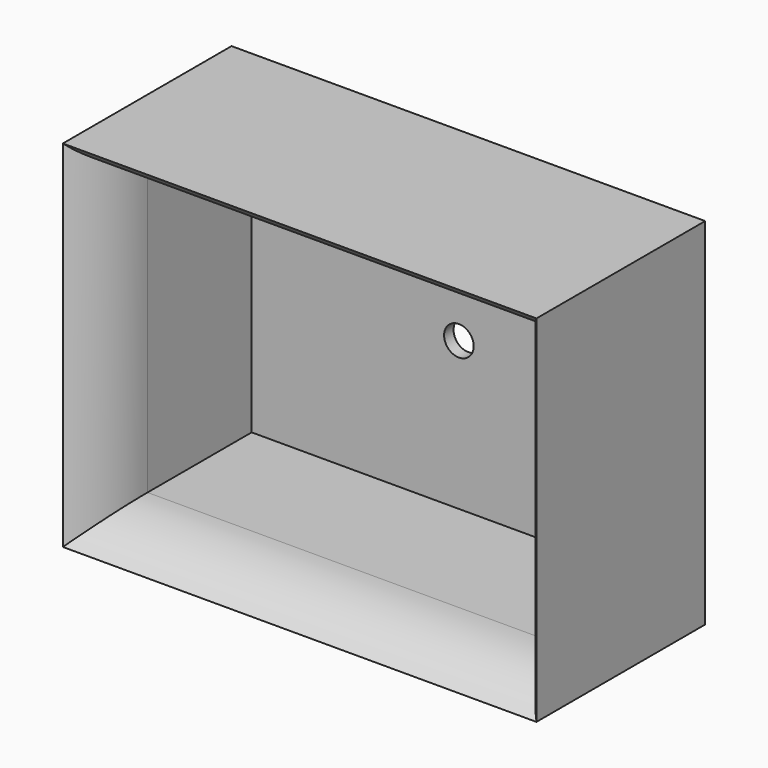
from build123d import *

# Parameters (mm, degrees)
F0_W         = 101.6
F0_H         = 76.2
F0_W_2       = 88.9
F0_H_2       = 63.5
F1_DEPTH     = 50.8
F2_DEPTH     = 2.54
F3_T1_DEPTH  = 63.5
F3_T3_DEPTH  = 88.9
F3_T9_DEPTH  = 139.7
F3_T15_DEPTH = 114.3
F3_T24_DEPTH = 139.7
F3_T30_DEPTH = 114.3
F3_T39_DEPTH = 139.7
F3_T45_DEPTH = 114.3
F3_T54_DEPTH = 114.3
F3_T60_DEPTH = 139.7
F4_R         = 3.175
F5_DEPTH     = 2.541


# Not quite as in the source:
# - a fillet or chamfer that OpenCascade refuses, or shapes differently, is made with other operations: its cross-section is extruded or revolved along the edge and cut away or added


with BuildPart() as f1:
    # F0 (on Front) → F1 (new body)
    with BuildSketch(Plane.XZ):
        Rectangle(F0_W, F0_H)
        Rectangle(F0_W_2, F0_H_2, mode=Mode.SUBTRACT)
    extrude(amount=F1_DEPTH)

    # F3: fillet of radius 20.32 on 4 edges, made by hand

    # F3_s2 → F3_t1 (cut)
    with BuildSketch(Plane.XY.offset(-31.75)):
        with BuildLine():
            ThreePointArc((-44.45, -30.48), (-50.4015902063, -44.8484097937), (-64.77, -50.8))
            Line((-64.77, -50.8), (-44.45, -50.8))
            Line((-44.45, -50.8), (-44.45, -30.48))
        make_face()
        with BuildLine():
            ThreePointArc((44.45, -30.48), (50.4015902063, -44.8484097937), (64.77, -50.8))
            Line((64.77, -50.8), (44.45, -50.8))
            Line((44.45, -50.8), (44.45, -30.48))
        make_face()
    extrude(amount=F3_T1_DEPTH, mode=Mode.SUBTRACT)

    # F3_s4 → F3_t3 (cut)
    with BuildSketch(Plane.YZ.offset(-44.45)):
        with BuildLine():
            ThreePointArc((-30.48, 31.75), (-44.8484097937, 37.7015902063), (-50.8, 52.07))
            Line((-50.8, 52.07), (-50.8, 31.75))
            Line((-50.8, 31.75), (-30.48, 31.75))
        make_face()
        with BuildLine():
            ThreePointArc((-30.48, -31.75), (-44.8484097937, -37.7015902063), (-50.8, -52.07))
            Line((-50.8, -52.07), (-50.8, -31.75))
            Line((-50.8, -31.75), (-30.48, -31.75))
        make_face()
    extrude(amount=F3_T3_DEPTH, mode=Mode.SUBTRACT)


with BuildPart() as f2:
    # F0 (on Front) → F2 (new body)
    with BuildSketch(Plane.XZ):
        Rectangle(F0_W_2, F0_H_2)
    extrude(amount=F2_DEPTH)

    # F4 (on face) → F5 (cut, through all)
    with BuildSketch(Plane.XZ.offset(2.54)):
        Circle(F4_R)
    extrude(amount=-F5_DEPTH, mode=Mode.SUBTRACT)


with BuildPart() as f3_tool7:
    # F3_s8 → F3_t9 (new body)
    with BuildSketch(Plane.YZ.offset(44.45)):
        with BuildLine():
            ThreePointArc((-30.48, -31.75), (-44.8484097937, -37.7015902063), (-50.8, -52.07))
            Line((-50.8, -52.07), (-50.8, -31.75))
            Line((-50.8, -31.75), (-30.48, -31.75))
        make_face()
    extrude(amount=-F3_T9_DEPTH)

    split(bisect_by=Plane.YZ.offset(-50.8), keep=Keep.TOP)

    split(bisect_by=Plane.XY.offset(-38.1), keep=Keep.TOP)

    split(bisect_by=Plane.YZ.offset(-44.45), keep=Keep.BOTTOM)


with BuildPart() as f3_tool13:
    # F3_s14 → F3_t15 (new body)
    with BuildSketch(Plane.XY.offset(-82.55)):
        with BuildLine():
            ThreePointArc((-44.45, -30.48), (-50.4015902063, -44.8484097937), (-64.77, -50.8))
            Line((-64.77, -50.8), (-44.45, -50.8))
            Line((-44.45, -50.8), (-44.45, -30.48))
        make_face()
    extrude(amount=F3_T15_DEPTH)

    split(bisect_by=Plane.YZ.offset(-50.8), keep=Keep.TOP)

    split(bisect_by=Plane.XY.offset(-38.1), keep=Keep.TOP)

    split(bisect_by=Plane.XY.offset(-31.75), keep=Keep.BOTTOM)


with BuildPart() as f3_tool7_1:
    add(f3_tool7.part)

    # F3_t19: intersect F3_tool13
    add(f3_tool13.part, mode=Mode.INTERSECT)


with BuildPart() as f1_1:
    add(f1.part)

    # F3_t5: cut F3_tool7
    add(f3_tool7_1.part, mode=Mode.SUBTRACT)


with BuildPart() as f3_tool22:
    # F3_s23 → F3_t24 (new body)
    with BuildSketch(Plane.YZ.offset(-95.25)):
        with BuildLine():
            ThreePointArc((-30.48, 31.75), (-44.8484097937, 37.7015902063), (-50.8, 52.07))
            Line((-50.8, 52.07), (-50.8, 31.75))
            Line((-50.8, 31.75), (-30.48, 31.75))
        make_face()
    extrude(amount=F3_T24_DEPTH)

    split(bisect_by=Plane.XY.offset(38.1), keep=Keep.BOTTOM)

    split(bisect_by=Plane.YZ.offset(-50.8), keep=Keep.TOP)

    split(bisect_by=Plane.YZ.offset(-44.45), keep=Keep.BOTTOM)


with BuildPart() as f3_tool28:
    # F3_s29 → F3_t30 (new body)
    with BuildSketch(Plane.XY.offset(-31.75)):
        with BuildLine():
            ThreePointArc((-44.45, -30.48), (-50.4015902063, -44.8484097937), (-64.77, -50.8))
            Line((-64.77, -50.8), (-44.45, -50.8))
            Line((-44.45, -50.8), (-44.45, -30.48))
        make_face()
    extrude(amount=F3_T30_DEPTH)

    split(bisect_by=Plane.XY.offset(38.1), keep=Keep.BOTTOM)

    split(bisect_by=Plane.YZ.offset(-50.8), keep=Keep.TOP)

    split(bisect_by=Plane.XY.offset(31.75), keep=Keep.TOP)


with BuildPart() as f3_tool22_1:
    add(f3_tool22.part)

    # F3_t34: intersect F3_tool28
    add(f3_tool28.part, mode=Mode.INTERSECT)


with BuildPart() as f1_2:
    add(f1_1.part)

    # F3_t20: cut F3_tool22
    add(f3_tool22_1.part, mode=Mode.SUBTRACT)


with BuildPart() as f3_tool37:
    # F3_s38 → F3_t39 (new body)
    with BuildSketch(Plane.YZ.offset(-44.45)):
        with BuildLine():
            ThreePointArc((-30.48, 31.75), (-44.8484097937, 37.7015902063), (-50.8, 52.07))
            Line((-50.8, 52.07), (-50.8, 31.75))
            Line((-50.8, 31.75), (-30.48, 31.75))
        make_face()
    extrude(amount=F3_T39_DEPTH)

    split(bisect_by=Plane.YZ.offset(50.8), keep=Keep.BOTTOM)

    split(bisect_by=Plane.XY.offset(38.1), keep=Keep.BOTTOM)

    split(bisect_by=Plane.YZ.offset(44.45), keep=Keep.TOP)


with BuildPart() as f3_tool43:
    # F3_s44 → F3_t45 (new body)
    with BuildSketch(Plane.XY.offset(82.55)):
        with BuildLine():
            ThreePointArc((44.45, -30.48), (50.4015902063, -44.8484097937), (64.77, -50.8))
            Line((64.77, -50.8), (44.45, -50.8))
            Line((44.45, -50.8), (44.45, -30.48))
        make_face()
    extrude(amount=-F3_T45_DEPTH)

    split(bisect_by=Plane.YZ.offset(50.8), keep=Keep.BOTTOM)

    split(bisect_by=Plane.XY.offset(38.1), keep=Keep.BOTTOM)

    split(bisect_by=Plane.XY.offset(31.75), keep=Keep.TOP)


with BuildPart() as f3_tool37_1:
    add(f3_tool37.part)

    # F3_t49: intersect F3_tool43
    add(f3_tool43.part, mode=Mode.INTERSECT)


with BuildPart() as f1_3:
    add(f1_2.part)

    # F3_t35: cut F3_tool37
    add(f3_tool37_1.part, mode=Mode.SUBTRACT)


with BuildPart() as f3_tool52:
    # F3_s53 → F3_t54 (new body)
    with BuildSketch(Plane.XY.offset(31.75)):
        with BuildLine():
            ThreePointArc((44.45, -30.48), (50.4015902063, -44.8484097937), (64.77, -50.8))
            Line((64.77, -50.8), (44.45, -50.8))
            Line((44.45, -50.8), (44.45, -30.48))
        make_face()
    extrude(amount=-F3_T54_DEPTH)

    split(bisect_by=Plane.YZ.offset(50.8), keep=Keep.BOTTOM)

    split(bisect_by=Plane.XY.offset(-38.1), keep=Keep.TOP)

    split(bisect_by=Plane.XY.offset(-31.75), keep=Keep.BOTTOM)


with BuildPart() as f3_tool58:
    # F3_s59 → F3_t60 (new body)
    with BuildSketch(Plane.YZ.offset(95.25)):
        with BuildLine():
            ThreePointArc((-30.48, -31.75), (-44.8484097937, -37.7015902063), (-50.8, -52.07))
            Line((-50.8, -52.07), (-50.8, -31.75))
            Line((-50.8, -31.75), (-30.48, -31.75))
        make_face()
    extrude(amount=-F3_T60_DEPTH)

    split(bisect_by=Plane.YZ.offset(50.8), keep=Keep.BOTTOM)

    split(bisect_by=Plane.XY.offset(-38.1), keep=Keep.TOP)

    split(bisect_by=Plane.YZ.offset(44.45), keep=Keep.TOP)


with BuildPart() as f3_tool52_1:
    add(f3_tool52.part)

    # F3_t64: intersect F3_tool58
    add(f3_tool58.part, mode=Mode.INTERSECT)


with BuildPart() as f1_4:
    add(f1_3.part)

    # F3_t50: cut F3_tool52
    add(f3_tool52_1.part, mode=Mode.SUBTRACT)


solid = Compound([f2.part, f1_4.part])
